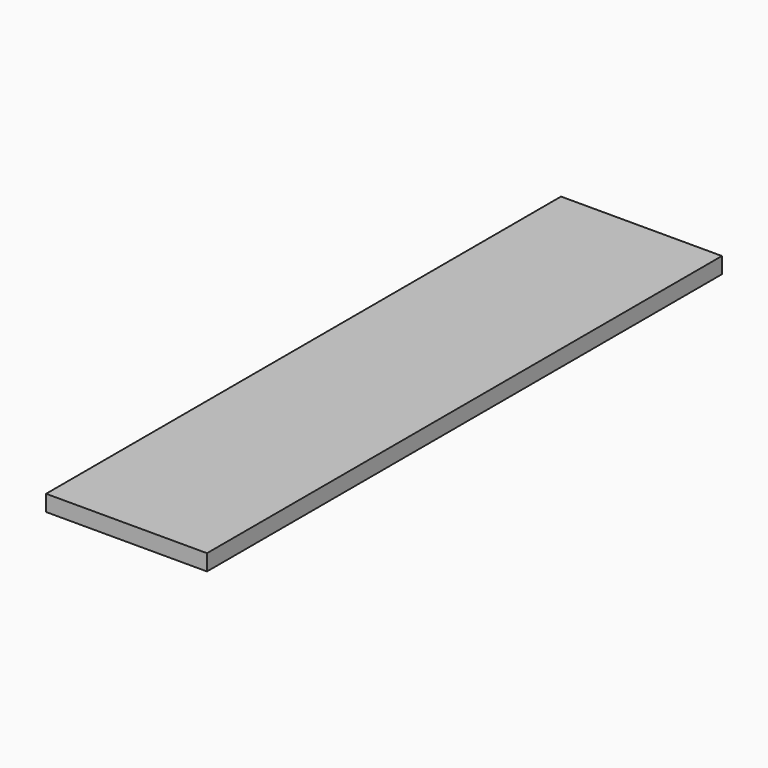
from build123d import *

# Parameters (mm, degrees)
F0_W     = 10
F0_H     = 1
F1_DEPTH = 40


# Not quite as in the source:
# - a feature names something its author has since deleted; it is built from what else it names


with BuildPart() as f1:
    # F0 (on Front) → F1 (new body)
    with BuildSketch(Plane.XZ):
        with Locations((4.5, 3)):
            Rectangle(F0_W, F0_H)
    extrude(amount=F1_DEPTH)


solid = f1.part
